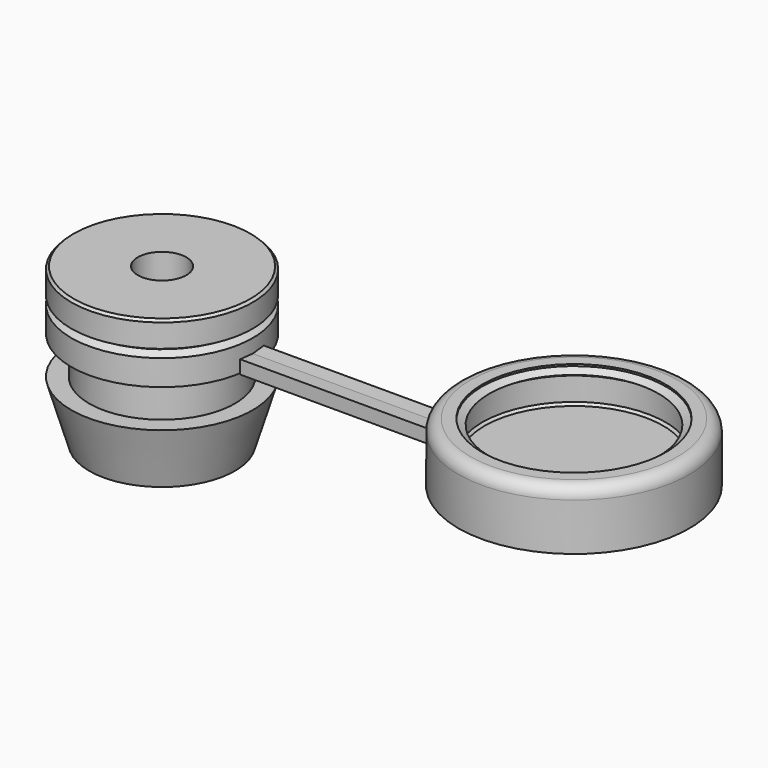
from build123d import *

# Parameters (mm, degrees)
F0_W         = 22.0345
F0_H         = 1.27
F3_DEPTH     = 1.5875
F3_TAPER     = -3
F4_SIZE      = 0.254
F5_R         = 1.27
F6_R         = 2.6035
F7_DEPTH     = 16.765
F8_TEXT_SIZE = 6.8712911646
F9_DEPTH     = 0.254


# Not quite as in the source:
# - a feature names something its author has since deleted; it is built from what else it names
# - Text() gives the source's letters only with a copy of the font that has no kerning and outlines rounded to 1/6400 em; it was checked with that copy


with BuildPart() as f1:
    # F0 (on Front) → F1 (revolve)
    with BuildSketch(Plane.XZ):
        Polygon((-7.8105, 0), (0, 0), (0, 16.764), (-9.7155, 16.764), (-9.7155, 14.0289409051), (-8.9535, 13.589), (-9.7155, 13.1490590949), (-9.7155, 10.414), (-7.8105, 10.414), (-7.8105, 6.35), (-9.7155, 6.35), align=None)
    revolve(axis=Axis((0, 0, 8.382), (0, 0, -1)))



with BuildPart() as f2:
    # F0 (on Front) → F2 (revolve)
    with BuildSketch(Plane.XZ):
        Polygon((34.2827288333, 16.764), (31.75, 16.764), (31.75, 11.684), (31.75, 10.414), (44.1252288333, 10.414), (44.1252288333, 12.954), (34.3045423334, 12.954), (34.3045423334, 15.6890590949), (35.0554013796, 16.1477558277), (34.2827288333, 16.56867047), align=None)
    revolve(axis=Axis((44.1252288333, 0, 11.684), (0, 0, -1)))


with BuildPart() as f1_1:
    add(f1.part)

    add(f2.part)  # F3 merges F2
    # F0 (on Front) → F3 (join, symmetric)
    with BuildSketch(Plane.XZ):
        with Locations((20.73275, 11.049)):
            Rectangle(F0_W, F0_H)
    extrude(amount=F3_DEPTH, both=True, taper=F3_TAPER)

    # F4
    f4_edges = [f1_1.edges().sort_by_distance(p)[0] for p in [
        (9.7155, 0, 16.764),
        (53.945915, 0, 12.954),
    ]]
    chamfer(f4_edges, length=F4_SIZE)

    # F5
    f5_edges = [f1_1.edges().sort_by_distance(p)[0] for p in [
        (56.500458, 0, 16.764),
    ]]
    fillet(f5_edges, radius=F5_R)

    # F6 (on face) → F7 (cut, through all)
    with BuildSketch(Plane(origin=(0, 0, 0), x_dir=(1, 0, 0), z_dir=(0, 0, -1))):
        Circle(F6_R)
    extrude(amount=-F7_DEPTH, mode=Mode.SUBTRACT)

    # F8 (on face) → F9 (cut)
    with BuildSketch(Plane(origin=(0, 0, 10.414), x_dir=(1, 0, 0), z_dir=(0, 0, -1))):
        with Locations((36.60216555, -1.6031591222)):
            Text('Vent', F8_TEXT_SIZE, font='Open Sans', text_align=(TextAlign.LEFT, TextAlign.BOTTOM))
    extrude(amount=-F9_DEPTH, mode=Mode.SUBTRACT)


solid = f1_1.part
